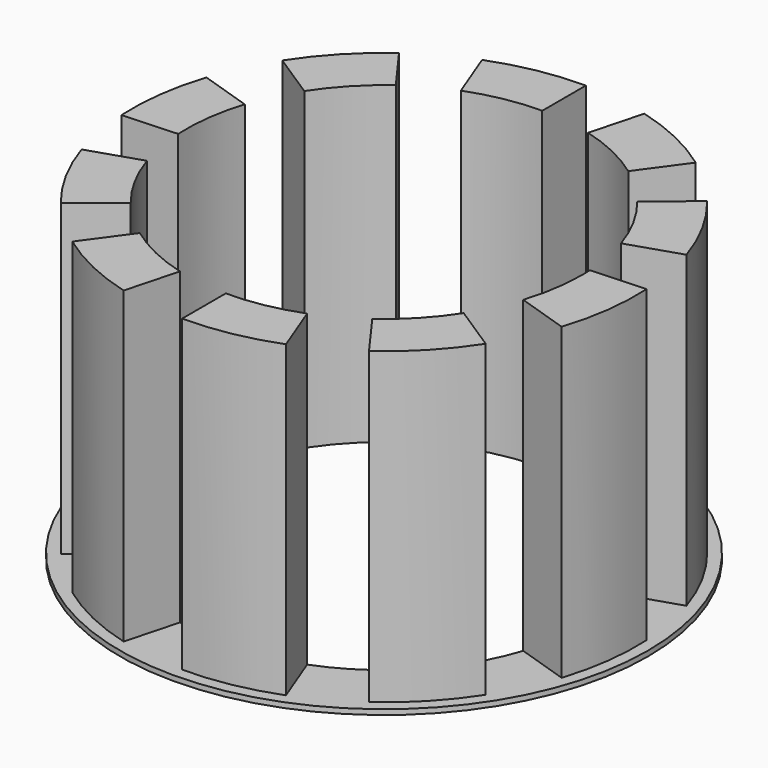
from build123d import *

# Parameters (mm, degrees)
F0_R            = 25.625
F1_DEPTH        = 0.5
F2_R            = 24.5
F3_DEPTH        = 30
F4_R            = 19.2
F5_DEPTH        = 30.501
F7_DEPTH        = 30
F7_COPIES_COUNT = 10


# Not quite as in the source:
# - a pattern or mirror of a feature is missing from the dataset's text; its kind, count and spacing are read off the source's solid


with BuildPart() as f1:
    # F0 (on Top) → F1 (new body)
    with BuildSketch(Plane.XY):
        Circle(F0_R)
    extrude(amount=F1_DEPTH)

    # F2 (on face) → F3 (join)
    with BuildSketch(Plane.XY.offset(0.5)):
        Circle(F2_R)
    extrude(amount=F3_DEPTH)

    # F4 (on face) → F5 (cut, through all)
    with BuildSketch(Plane.XY.offset(30.5)):
        Circle(F4_R)
    extrude(amount=-F5_DEPTH, mode=Mode.SUBTRACT)

    # F6 (on face) → F7 (cut, through all)
    with BuildSketch(Plane.XY.offset(30.5)):
        with BuildLine():
            Line((4.969325666, 18.5457758648), (6.341066605, 23.6651827441))
            ThreePointArc((6.341066605, 23.6651827441), (3.1978917094, 24.2903991037), (0, 24.5))
            Line((0, 24.5), (0, 19.2))
            ThreePointArc((0, 19.2), (2.5061028906, 19.0357413384), (4.969325666, 18.5457758648))
        make_face()
    f7 = extrude(amount=-F7_DEPTH, mode=Mode.SUBTRACT)

    # F7_copies: F7 ×10 about axis
    f7_copies_axis = Axis((0, 0, 0), (0, 0, 1))
    for i in range(1, F7_COPIES_COUNT):
        add(f7.rotate(f7_copies_axis, i * 360 / F7_COPIES_COUNT), mode=Mode.SUBTRACT)


solid = f1.part
